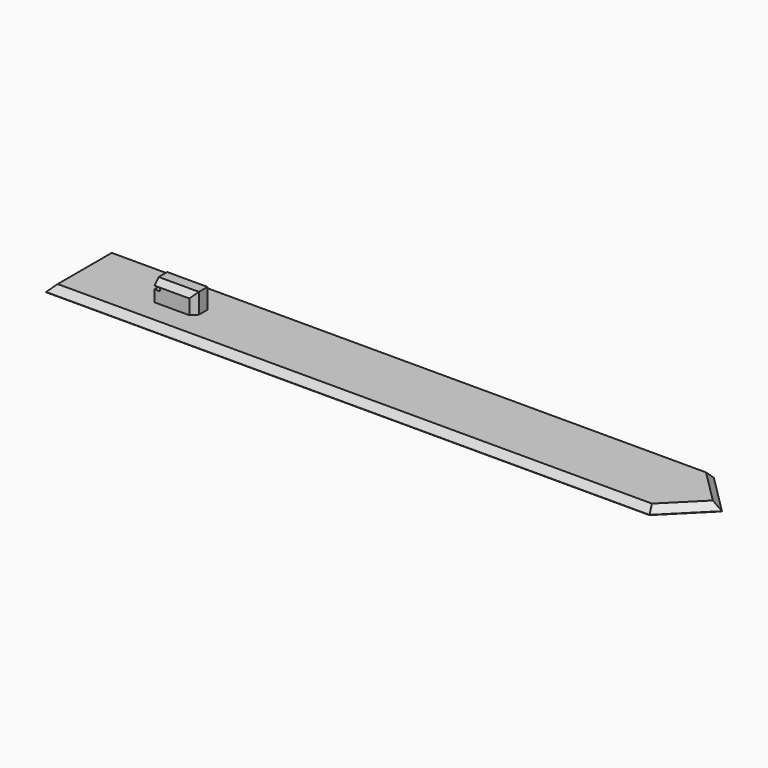
from build123d import *

# Parameters (mm, degrees)
F0_W         = 152.4
F0_H         = 19.05
F1_DEPTH     = 1.5875
F2_SIZE      = 9.52499
F3_W         = 9.525
F3_H         = 5.08
F4_DEPTH     = 4.7625
F5_SIZE      = 1.27
F6_W         = 5.08
F6_H         = 0.762
F7_DEPTH     = 1.27
F8_SIZE      = 1.524
F9_T1_DEPTH  = 19.1535983177
F9_T3_DEPTH  = 7.8385097473
F9_T5_DEPTH  = 21.3088597868
F9_T7_DEPTH  = 150.7134997473
F9_T9_DEPTH  = 25.3644897473
F9_T14_DEPTH = 9.4899593576
F9_T19_DEPTH = 9.4899593576
F9_T24_DEPTH = 9.4899593576
F9_T29_DEPTH = 9.4899593576


# Not quite as in the source:
# - a fillet or chamfer that OpenCascade refuses, or shapes differently, is made with other operations: its cross-section is extruded or revolved along the edge and cut away or added
# - two fillets or chamfers of one size are made in one step
# - a fillet or chamfer is up to 0.001 mm smaller than in the source, because OpenCascade refuses the exact size


with BuildPart() as f1:
    # F0 (on Top) → F1 (new body)
    with BuildSketch(Plane.XY):
        with Locations((2.4961568415, 22.6473969003)):
            Rectangle(F0_W, F0_H)
    extrude(amount=-F1_DEPTH)

    # F2 (size 9.525 in the source; OpenCascade refuses exactly that, so slightly less here)
    f2_edges = [f1.edges().sort_by_distance(p)[0] for p in [
        (78.696157, 13.122397, -0.79375),
        (78.696157, 32.172397, -0.79375),
    ]]
    chamfer(f2_edges, length=F2_SIZE)

    # F3 (on face) → F4 (join)
    with BuildSketch(Plane.XY):
        with Locations((-48.8753431585, 22.6473969003)):
            Rectangle(F3_W, F3_H)
    extrude(amount=F4_DEPTH)

    # F5
    f5_edges = [f1.edges().sort_by_distance(p)[0] for p in [
        (-44.112843, 20.107397, 2.38125),
        (-44.112843, 25.187397, 2.38125),
        (-48.875343, 25.187397, 4.7625),
        (-48.875343, 20.107397, 4.7625),
    ]]
    chamfer(f5_edges, length=F5_SIZE)

    # F6 (on face) → F7 (cut)
    with BuildSketch(Plane(origin=(-53.6378431585, 0, 0), x_dir=(0, -1, 0), z_dir=(-1, 0, 0))):
        with Locations((-22.6473969003, 3.1115)):
            Rectangle(F6_W, F6_H)
    extrude(amount=-F7_DEPTH, mode=Mode.SUBTRACT)

    # F8
    f8_edges = [f1.edges().sort_by_distance(p)[0] for p in [
        (-2.266338, 13.122397, 0),
    ]]
    chamfer(f8_edges, length=F8_SIZE)

    # F9: chamfer of 1.524 on 7 edges, made by hand

    # F9_s2 → F9_t1 (cut)
    with BuildSketch(Plane(origin=(53.4430964982, 53.4430964982, 0), x_dir=(0, 0, 1), z_dir=(-0.7071067812, -0.7071067812, 0))):
        Polygon((0, -38.1084653026), (-1.524, -39.6324653026), (0, -39.6324653026), align=None)
    extrude(amount=F9_T1_DEPTH, mode=Mode.SUBTRACT)

    # F9_s4 → F9_t3 (cut)
    with BuildSketch(Plane.XZ.offset(-26.566651774)):
        Polygon((77.1721568415, 0), (78.6961568415, -1.524), (78.6961568415, 0), align=None)
    extrude(amount=F9_T3_DEPTH, mode=Mode.SUBTRACT)

    # F9_s6 → F9_t5 (cut)
    with BuildSketch(Plane(origin=(30.7956995979, -30.7956995979, 0), x_dir=(0, 0, 1), z_dir=(-0.7071067812, 0.7071067812, 0))):
        Polygon((0, 70.1367211515), (-1.524, 71.6607211515), (0, 71.6607211515), align=None)
    extrude(amount=F9_T5_DEPTH, mode=Mode.SUBTRACT)

    # F9_s8 → F9_t7 (cut)
    with BuildSketch(Plane.YZ.offset(-77.6230880321)):
        Polygon((30.6483969003, 0), (32.1723969003, -1.524), (32.1723969003, 0), align=None)
    extrude(amount=F9_T7_DEPTH, mode=Mode.SUBTRACT)

    # F9_s10 → F9_t9 (cut)
    with BuildSketch(Plane.XZ.offset(-36.091641774)):
        Polygon((-72.1798431585, 0), (-73.7038431585, -1.524), (-73.7038431585, 0), align=None)
    extrude(amount=F9_T9_DEPTH, mode=Mode.SUBTRACT)


with BuildPart() as f9_tool12:
    # F9_s13 → F9_t14 (new body)
    with BuildSketch(Plane.XY.offset(3.9512296788)):
        Polygon((77.618526107, 21.5697561658), (78.6961568415, 24.1713869003), (78.6961568415, 22.6473869003), align=None)
    extrude(amount=-F9_T14_DEPTH)

    split(bisect_by=Plane(origin=(38.5860784208, 0, 38.5860784208), x_dir=(0, 1, 0), z_dir=(0.7071067812, 0, 0.7071067812)), keep=Keep.TOP)


with BuildPart() as f1_1:
    add(f1.part)

    # F9_t11: cut F9_tool12
    add(f9_tool12.part, mode=Mode.SUBTRACT)


with BuildPart() as f9_tool17:
    # F9_s18 → F9_t19 (new body)
    with BuildSketch(Plane.XY.offset(3.9512296788)):
        Polygon((77.618526107, 21.5697561658), (78.6961568415, 24.1713869003), (78.6961568415, 22.6473869003), align=None)
    extrude(amount=-F9_T19_DEPTH)

    split(bisect_by=Plane(origin=(13.473377118, -13.473377118, 19.0542326513), x_dir=(0.7071067812, 0.7071067812, 0), z_dir=(0.5, -0.5, 0.7071067812)), keep=Keep.TOP)


with BuildPart() as f1_2:
    add(f1_1.part)

    # F9_t16: cut F9_tool17
    add(f9_tool17.part, mode=Mode.SUBTRACT)


with BuildPart() as f9_tool22:
    # F9_s23 → F9_t24 (new body)
    with BuildSketch(Plane.XY.offset(3.9512296788)):
        Polygon((78.6961568415, 21.1234069003), (77.618526107, 23.7250376349), (78.6961568415, 22.6474069003), align=None)
    extrude(amount=-F9_T24_DEPTH)

    split(bisect_by=Plane(origin=(24.7970755682, 24.7970755682, 35.0683605757), x_dir=(-0.7071067812, 0.7071067812, 0), z_dir=(0.5, 0.5, 0.7071067812)), keep=Keep.TOP)


with BuildPart() as f1_3:
    add(f1_2.part)

    # F9_t21: cut F9_tool22
    add(f9_tool22.part, mode=Mode.SUBTRACT)


with BuildPart() as f9_tool27:
    # F9_s28 → F9_t29 (new body)
    with BuildSketch(Plane.XY.offset(3.9512296788)):
        Polygon((78.6961568415, 21.1234069003), (77.618526107, 23.7250376349), (78.6961568415, 22.6474069003), align=None)
    extrude(amount=-F9_T29_DEPTH)

    split(bisect_by=Plane(origin=(38.5860784208, 0, 38.5860784208), x_dir=(0, 1, 0), z_dir=(0.7071067812, 0, 0.7071067812)), keep=Keep.TOP)


with BuildPart() as f1_4:
    add(f1_3.part)

    # F9_t26: cut F9_tool27
    add(f9_tool27.part, mode=Mode.SUBTRACT)


solid = f1_4.part
